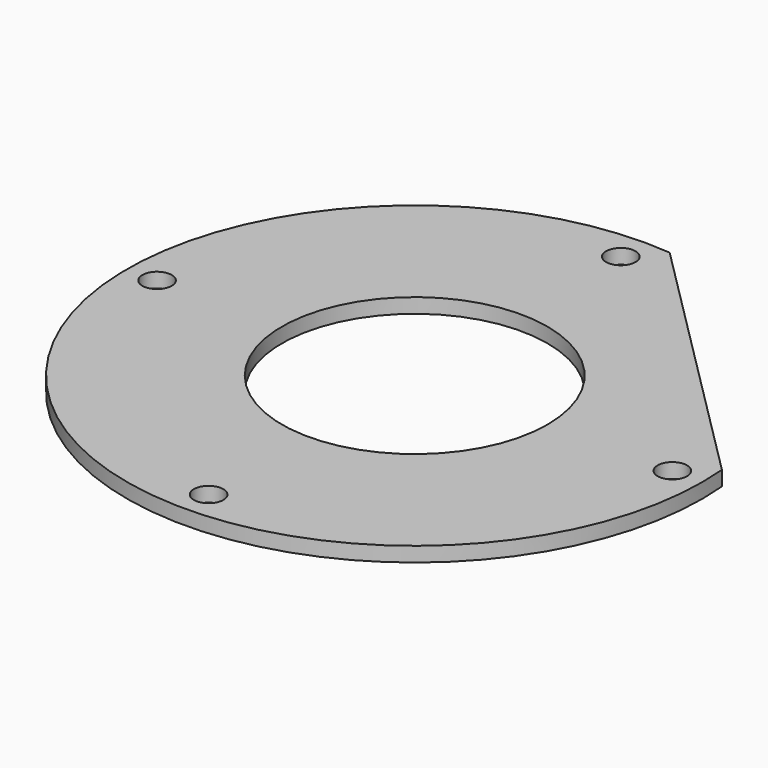
from build123d import *

# Parameters (mm, degrees)
F0_R     = 97.79
F0_R_2   = 5
F0_R_3   = 45.085
F1_DEPTH = 5
F3_DEPTH = 5.001


# Not quite as in the source:
# - a feature names something its author has since deleted; it is built from what else it names


with BuildPart() as f1:
    # F0 (on Top) → F1 (new body)
    with BuildSketch(Plane.XY):
        Circle(F0_R)
        with Locations((0, -87.5)):
            Circle(F0_R_2, mode=Mode.SUBTRACT)
        with Locations((-87.5, 0)):
            Circle(F0_R_2, mode=Mode.SUBTRACT)
        Circle(F0_R_3, mode=Mode.SUBTRACT)
        with Locations((87.5, 0)):
            Circle(F0_R_2, mode=Mode.SUBTRACT)
        with Locations((0, 87.5)):
            Circle(F0_R_2, mode=Mode.SUBTRACT)
    extrude(amount=F1_DEPTH)

    # F2 (on face) → F3 (cut, through all)
    with BuildSketch(Plane.XY.offset(5)):
        with BuildLine():
            ThreePointArc((97.4057710678, 8.6602461102), (69.1479721322, 69.1479721322), (8.6602461102, 97.4057710678))
            Line((8.6602461102, 97.4057710678), (97.4057710678, 8.6602461102))
        make_face()
    extrude(amount=-F3_DEPTH, mode=Mode.SUBTRACT)


solid = f1.part
